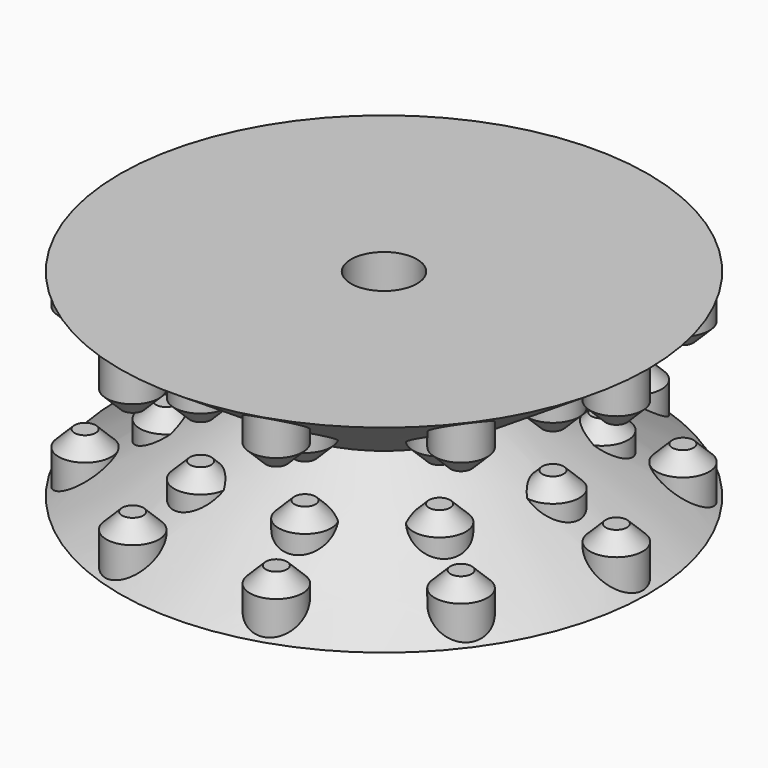
from build123d import *

# Parameters (mm, degrees)
F0_R      = 12.7
F2_R      = 5.4465248762
F5_R      = 1.27
F6_DEPTH  = 1.27
F10_R     = 1.27
F11_DEPTH = 1.778
F13_COUNT = 10
F14_R     = 1.5875
F15_DEPTH = 4.7635001


# Not quite as in the source:
# - a fillet or chamfer that OpenCascade refuses, or shapes differently, is made with other operations: its cross-section is extruded or revolved along the edge and cut away or added


with BuildPart() as f3:
    # F0 (on Top) → F3 section 0
    with BuildSketch(Plane.XY):
        with Locations((-15.2407279238, 5.2362736315)):
            Circle(F0_R)
    # F2 (on offset) → F3 section 1
    with BuildSketch(Plane.XY.offset(4.7625)):
        with Locations((-15.2407279238, 5.2362736315)):
            Circle(F2_R)
    loft()

    # F5 (on offset) → F6 (join, symmetric)
    with BuildSketch(Plane(origin=(0, 0, 1.27), x_dir=(1, 0, 0), z_dir=(0, 0, -1))):
        with Locations((-4.0008900687, -5.1531763747)):
            Circle(F5_R)
    extrude(amount=F6_DEPTH, both=True)

    # F7: chamfer of 0.762 on 1 edges, made by hand

    # F7_s1 → F7_t2 (revolve, cut)
    with BuildSketch(Plane.XZ.offset(-5.1531763747)):
        with BuildLine():
            Line((-2.709337454, 1.7564473853), (-3.5144426834, 2.5615526147))
            Line((-3.5144426834, 2.5615526147), (-3.5144426834, 2.5767926147))
            ThreePointArc((-3.5144426834, 2.5767926147), (-3.1226663761, 2.55524), (-2.7308900687, 2.55524))
            Line((-2.7308900687, 2.55524), (-2.7156500687, 2.54))
            ThreePointArc((-2.7156500687, 2.54), (-2.7156500687, 2.1482236927), (-2.694097454, 1.7564473853))
            Line((-2.694097454, 1.7564473853), (-2.709337454, 1.7564473853))
        make_face()
    revolve(axis=Axis((-4.0008900687, 5.1531763747, 2.54), (0, 0, -1)), mode=Mode.SUBTRACT)

    # F10 (on offset) → F11 (join)
    with BuildSketch(Plane(origin=(0, 0, 3.81), x_dir=(1, 0, 0), z_dir=(0, 0, -1))):
        with Locations((-7.0517784916, -5.1531763747)):
            Circle(F10_R)
    extrude(amount=F11_DEPTH)

    # F12: chamfer of 0.762 on 1 edges, made by hand

    # F12_s1 → F12_t2 (revolve, cut)
    with BuildSketch(Plane.XZ.offset(-5.1531763747)):
        with BuildLine():
            Line((-5.7602258769, 3.0264473853), (-6.5653311063, 3.8315526147))
            Line((-6.5653311063, 3.8315526147), (-6.5653311063, 3.8467926147))
            ThreePointArc((-6.5653311063, 3.8467926147), (-6.1735547989, 3.82524), (-5.7817784916, 3.82524))
            Line((-5.7817784916, 3.82524), (-5.7665384916, 3.81))
            ThreePointArc((-5.7665384916, 3.81), (-5.7665384916, 3.4182236927), (-5.7449858769, 3.0264473853))
            Line((-5.7449858769, 3.0264473853), (-5.7602258769, 3.0264473853))
        make_face()
    revolve(axis=Axis((-7.0517784916, 5.1531763747, 3.81), (0, 0, -1)), mode=Mode.SUBTRACT)

    # F13: F3 ×10 about axis
    f13_axis = Axis((-15.2407279238, 5.2362736315, 0), (0, 0, 1))


with BuildPart() as f3_1:
    add(f3.part)
    for i in range(1, F13_COUNT):
        add(f3.part.rotate(f13_axis, i * 360 / F13_COUNT))

    # F14 (on face) → F15 (cut, through all)
    with BuildSketch(Plane.XY.offset(4.7625)):
        with Locations((-15.2407279238, 5.2362736315)):
            Circle(F14_R)
    extrude(amount=-F15_DEPTH, mode=Mode.SUBTRACT)

    # F16: F3 across face


with BuildPart() as f3_2:
    add(f3_1.part)
    add(f3_1.part.mirror(Plane.XY.offset(4.7625)))


solid = f3_2.part
